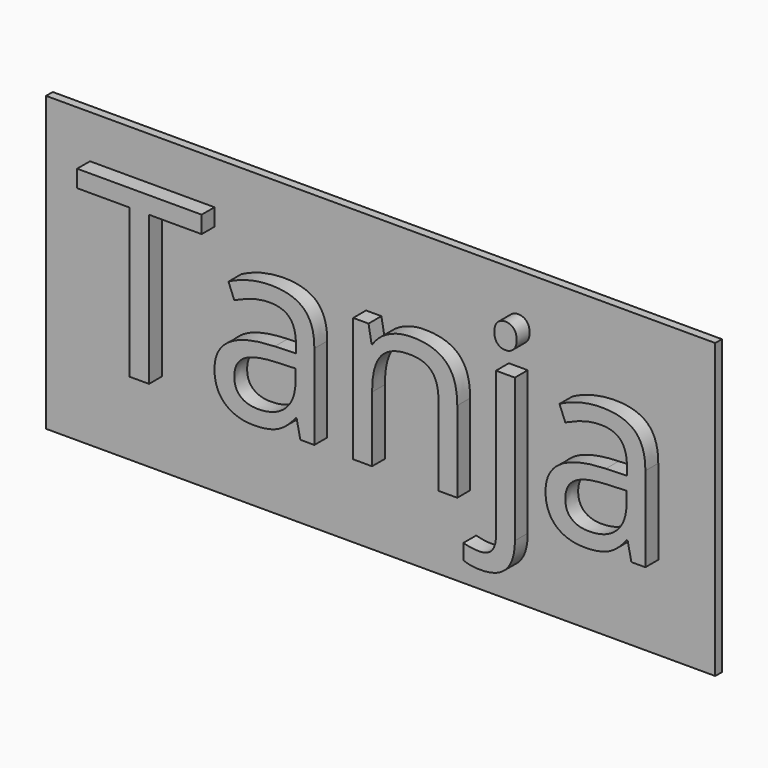
from build123d import *

# Parameters (mm, degrees)
F0_TEXT_SIZE = 27.7777777778
F1_DEPTH     = 2.920278348
F0_W         = 79.8914930556
F0_H         = 35
F2_DEPTH     = 1


# Not quite as in the source:
# - Text() gives the source's letters only with a copy of the font that has no kerning and outlines rounded to 1/6400 em; it was checked with that copy


with BuildPart() as f1:
    # F0 (on Front) → F1 (new body)
    with BuildSketch(Plane.XZ):
        with Locations((0, 0)):
            Text('Tanja', F0_TEXT_SIZE, font='Open Sans', text_align=(TextAlign.LEFT, TextAlign.BOTTOM))
    extrude(amount=F1_DEPTH)

    # F0 (on Front) → F2 (join)
    with BuildSketch(Plane.XZ):
        with Locations((34.9457465278, 7.5)):
            Rectangle(F0_W, F0_H)
        with BuildLine():
            Line((28.5677083333, 0), (26.8967013889, 0))
            Line((26.8967013889, 0), (26.4496527778, 2.1180555556))
            Line((26.4496527778, 2.1180555556), (26.3411458333, 2.1180555556))
            add(Edge.make_bspline(
                [(26.3411458333, 2.1180555556), (25.2300347222, 0.7204861111), (24.1254340278, 0.2235243056)],
                knots=[0, 0, 0, 1, 1, 1], degree=2))
            add(Edge.make_bspline(
                [(24.1254340278, 0.2235243056), (23.0208333333, -0.2734375), (21.3628472222, -0.2734375)],
                knots=[0, 0, 0, 1, 1, 1], degree=2))
            add(Edge.make_bspline(
                [(21.3628472222, -0.2734375), (19.1536458333, -0.2734375), (17.8993055556, 0.8680555556)],
                knots=[0, 0, 0, 1, 1, 1], degree=2))
            add(Edge.make_bspline(
                [(17.8993055556, 0.8680555556), (16.6449652778, 2.0095486111), (16.6449652778, 4.1102430556)],
                knots=[0, 0, 0, 1, 1, 1], degree=2))
            add(Edge.make_bspline(
                [(16.6449652778, 4.1102430556), (16.6449652778, 8.6111111111), (23.8454861111, 8.828125)],
                knots=[0, 0, 0, 1, 1, 1], degree=2))
            Line((23.8454861111, 8.828125), (26.3671875, 8.9105902778))
            Line((26.3671875, 8.9105902778), (26.3671875, 9.8350694444))
            add(Edge.make_bspline(
                [(26.3671875, 9.8350694444), (26.3671875, 11.5842013889), (25.6163194444, 12.4175347222)],
                knots=[0, 0, 0, 1, 1, 1], degree=2))
            add(Edge.make_bspline(
                [(25.6163194444, 12.4175347222), (24.8654513889, 13.2508680556), (23.2074652778, 13.2508680556)],
                knots=[0, 0, 0, 1, 1, 1], degree=2))
            add(Edge.make_bspline(
                [(23.2074652778, 13.2508680556), (21.3498263889, 13.2508680556), (19.0060763889, 12.1137152778)],
                knots=[0, 0, 0, 1, 1, 1], degree=2))
            Line((19.0060763889, 12.1137152778), (18.3116319444, 13.8368055556))
            add(Edge.make_bspline(
                [(18.3116319444, 13.8368055556), (19.4097222222, 14.4314236111), (20.7183159722, 14.7699652778)],
                knots=[0, 0, 0, 1, 1, 1], degree=2))
            add(Edge.make_bspline(
                [(20.7183159722, 14.7699652778), (22.0269097222, 15.1085069444), (23.3463541667, 15.1085069444)],
                knots=[0, 0, 0, 1, 1, 1], degree=2))
            add(Edge.make_bspline(
                [(23.3463541667, 15.1085069444), (26.0026041667, 15.1085069444), (27.28515625, 13.9301215278)],
                knots=[0, 0, 0, 1, 1, 1], degree=2))
            add(Edge.make_bspline(
                [(27.28515625, 13.9301215278), (28.5677083333, 12.7517361111), (28.5677083333, 10.1475694444)],
                knots=[0, 0, 0, 1, 1, 1], degree=2))
            Line((28.5677083333, 10.1475694444), (28.5677083333, 0))
        make_face(mode=Mode.SUBTRACT)
        with BuildLine():
            add(Edge.make_bspline(
                [(52.5043402778, -2.2786458333), (52.5043402778, -6.6753472222), (48.4461805556, -6.6753472222)],
                knots=[0, 0, 0, 1, 1, 1], degree=2))
            add(Edge.make_bspline(
                [(48.4461805556, -6.6753472222), (47.1571180556, -6.6753472222), (46.3585069444, -6.3324652778)],
                knots=[0, 0, 0, 1, 1, 1], degree=2))
            Line((46.3585069444, -6.3324652778), (46.3585069444, -4.5052083333))
            add(Edge.make_bspline(
                [(46.3585069444, -4.5052083333), (47.2960069444, -4.7743055556), (48.203125, -4.7743055556)],
                knots=[0, 0, 0, 1, 1, 1], degree=2))
            add(Edge.make_bspline(
                [(48.203125, -4.7743055556), (49.2621527778, -4.7743055556), (49.7569444444, -4.1970486111)],
                knots=[0, 0, 0, 1, 1, 1], degree=2))
            add(Edge.make_bspline(
                [(49.7569444444, -4.1970486111), (50.2517361111, -3.6197916667), (50.2517361111, -2.4435763889)],
                knots=[0, 0, 0, 1, 1, 1], degree=2))
            Line((50.2517361111, -2.4435763889), (50.2517361111, 14.8654513889))
            Line((50.2517361111, 14.8654513889), (52.5043402778, 14.8654513889))
            Line((52.5043402778, 14.8654513889), (52.5043402778, -2.2786458333))
        make_face(mode=Mode.SUBTRACT)
        with BuildLine():
            Line((68.0902777778, 0), (66.4192708333, 0))
            Line((66.4192708333, 0), (65.9722222222, 2.1180555556))
            Line((65.9722222222, 2.1180555556), (65.8637152778, 2.1180555556))
            add(Edge.make_bspline(
                [(65.8637152778, 2.1180555556), (64.7526041667, 0.7204861111), (63.6480034722, 0.2235243056)],
                knots=[0, 0, 0, 1, 1, 1], degree=2))
            add(Edge.make_bspline(
                [(63.6480034722, 0.2235243056), (62.5434027778, -0.2734375), (60.8854166667, -0.2734375)],
                knots=[0, 0, 0, 1, 1, 1], degree=2))
            add(Edge.make_bspline(
                [(60.8854166667, -0.2734375), (58.6762152778, -0.2734375), (57.421875, 0.8680555556)],
                knots=[0, 0, 0, 1, 1, 1], degree=2))
            add(Edge.make_bspline(
                [(57.421875, 0.8680555556), (56.1675347222, 2.0095486111), (56.1675347222, 4.1102430556)],
                knots=[0, 0, 0, 1, 1, 1], degree=2))
            add(Edge.make_bspline(
                [(56.1675347222, 4.1102430556), (56.1675347222, 8.6111111111), (63.3680555556, 8.828125)],
                knots=[0, 0, 0, 1, 1, 1], degree=2))
            Line((63.3680555556, 8.828125), (65.8897569444, 8.9105902778))
            Line((65.8897569444, 8.9105902778), (65.8897569444, 9.8350694444))
            add(Edge.make_bspline(
                [(65.8897569444, 9.8350694444), (65.8897569444, 11.5842013889), (65.1388888889, 12.4175347222)],
                knots=[0, 0, 0, 1, 1, 1], degree=2))
            add(Edge.make_bspline(
                [(65.1388888889, 12.4175347222), (64.3880208333, 13.2508680556), (62.7300347222, 13.2508680556)],
                knots=[0, 0, 0, 1, 1, 1], degree=2))
            add(Edge.make_bspline(
                [(62.7300347222, 13.2508680556), (60.8723958333, 13.2508680556), (58.5286458333, 12.1137152778)],
                knots=[0, 0, 0, 1, 1, 1], degree=2))
            Line((58.5286458333, 12.1137152778), (57.8342013889, 13.8368055556))
            add(Edge.make_bspline(
                [(57.8342013889, 13.8368055556), (58.9322916667, 14.4314236111), (60.2408854167, 14.7699652778)],
                knots=[0, 0, 0, 1, 1, 1], degree=2))
            add(Edge.make_bspline(
                [(60.2408854167, 14.7699652778), (61.5494791667, 15.1085069444), (62.8689236111, 15.1085069444)],
                knots=[0, 0, 0, 1, 1, 1], degree=2))
            add(Edge.make_bspline(
                [(62.8689236111, 15.1085069444), (65.5251736111, 15.1085069444), (66.8077256944, 13.9301215278)],
                knots=[0, 0, 0, 1, 1, 1], degree=2))
            add(Edge.make_bspline(
                [(66.8077256944, 13.9301215278), (68.0902777778, 12.7517361111), (68.0902777778, 10.1475694444)],
                knots=[0, 0, 0, 1, 1, 1], degree=2))
            Line((68.0902777778, 10.1475694444), (68.0902777778, 0))
        make_face(mode=Mode.SUBTRACT)
        Polygon((8.828125, 17.7821180556), (8.828125, 0), (6.5234375, 0), (6.5234375, 17.7821180556), (0.2430555556, 17.7821180556), (0.2430555556, 19.8307291667), (15.1085069444, 19.8307291667), (15.1085069444, 17.7821180556), align=None, mode=Mode.SUBTRACT)
        with BuildLine():
            Line((45.6293402778, 0), (43.3767361111, 0))
            Line((43.3767361111, 0), (43.3767361111, 9.6180555556))
            add(Edge.make_bspline(
                [(43.3767361111, 9.6180555556), (43.3767361111, 11.4322916667), (42.5499131944, 12.3285590278)],
                knots=[0, 0, 0, 1, 1, 1], degree=2))
            add(Edge.make_bspline(
                [(42.5499131944, 12.3285590278), (41.7230902778, 13.2248263889), (39.9565972222, 13.2248263889)],
                knots=[0, 0, 0, 1, 1, 1], degree=2))
            add(Edge.make_bspline(
                [(39.9565972222, 13.2248263889), (37.6258680556, 13.2248263889), (36.5407986111, 11.9639756944)],
                knots=[0, 0, 0, 1, 1, 1], degree=2))
            add(Edge.make_bspline(
                [(36.5407986111, 11.9639756944), (35.4557291667, 10.703125), (35.4557291667, 7.7994791667)],
                knots=[0, 0, 0, 1, 1, 1], degree=2))
            Line((35.4557291667, 7.7994791667), (35.4557291667, 0))
            Line((35.4557291667, 0), (33.203125, 0))
            Line((33.203125, 0), (33.203125, 14.8654513889))
            Line((33.203125, 14.8654513889), (35.0347222222, 14.8654513889))
            Line((35.0347222222, 14.8654513889), (35.3993055556, 12.8298611111))
            Line((35.3993055556, 12.8298611111), (35.5078125, 12.8298611111))
            add(Edge.make_bspline(
                [(35.5078125, 12.8298611111), (36.2022569444, 13.9279513889), (37.4500868056, 14.5334201389)],
                knots=[0, 0, 0, 1, 1, 1], degree=2))
            add(Edge.make_bspline(
                [(37.4500868056, 14.5334201389), (38.6979166667, 15.1388888889), (40.2300347222, 15.1388888889)],
                knots=[0, 0, 0, 1, 1, 1], degree=2))
            add(Edge.make_bspline(
                [(40.2300347222, 15.1388888889), (42.9166666667, 15.1388888889), (44.2730034722, 13.8433159722)],
                knots=[0, 0, 0, 1, 1, 1], degree=2))
            add(Edge.make_bspline(
                [(44.2730034722, 13.8433159722), (45.6293402778, 12.5477430556), (45.6293402778, 9.6961805556)],
                knots=[0, 0, 0, 1, 1, 1], degree=2))
            Line((45.6293402778, 9.6961805556), (45.6293402778, 0))
        make_face(mode=Mode.SUBTRACT)
        with BuildLine():
            add(Edge.make_bspline(
                [(50.4405381944, 17.7604166667), (50.0607638889, 18.1336805556), (50.0607638889, 18.8932291667)],
                knots=[0, 0, 0, 1, 1, 1], degree=2))
            add(Edge.make_bspline(
                [(50.0607638889, 18.8932291667), (50.0607638889, 19.6657986111), (50.4405381944, 20.0260416667)],
                knots=[0, 0, 0, 1, 1, 1], degree=2))
            add(Edge.make_bspline(
                [(50.4405381944, 20.0260416667), (50.8203125, 20.3862847222), (51.3932291667, 20.3862847222)],
                knots=[0, 0, 0, 1, 1, 1], degree=2))
            add(Edge.make_bspline(
                [(51.3932291667, 20.3862847222), (51.9357638889, 20.3862847222), (52.3285590278, 20.01953125)],
                knots=[0, 0, 0, 1, 1, 1], degree=2))
            add(Edge.make_bspline(
                [(52.3285590278, 20.01953125), (52.7213541667, 19.6527777778), (52.7213541667, 18.8932291667)],
                knots=[0, 0, 0, 1, 1, 1], degree=2))
            add(Edge.make_bspline(
                [(52.7213541667, 18.8932291667), (52.7213541667, 18.1336805556), (52.3285590278, 17.7604166667)],
                knots=[0, 0, 0, 1, 1, 1], degree=2))
            add(Edge.make_bspline(
                [(52.3285590278, 17.7604166667), (51.9357638889, 17.3871527778), (51.3932291667, 17.3871527778)],
                knots=[0, 0, 0, 1, 1, 1], degree=2))
            add(Edge.make_bspline(
                [(51.3932291667, 17.3871527778), (50.8203125, 17.3871527778), (50.4405381944, 17.7604166667)],
                knots=[0, 0, 0, 1, 1, 1], degree=2))
        make_face(mode=Mode.SUBTRACT)
        with BuildLine():
            add(Edge.make_bspline(
                [(59.2664930556, 2.2243923611), (60.0043402778, 1.5885416667), (61.3324652778, 1.5885416667)],
                knots=[0, 0, 0, 1, 1, 1], degree=2))
            add(Edge.make_bspline(
                [(61.3324652778, 1.5885416667), (63.4375, 1.5885416667), (64.6375868056, 2.7408854167)],
                knots=[0, 0, 0, 1, 1, 1], degree=2))
            add(Edge.make_bspline(
                [(64.6375868056, 2.7408854167), (65.8376736111, 3.8932291667), (65.8376736111, 5.9678819444)],
                knots=[0, 0, 0, 1, 1, 1], degree=2))
            Line((65.8376736111, 5.9678819444), (65.8376736111, 7.3090277778))
            Line((65.8376736111, 7.3090277778), (63.5850694444, 7.2178819444))
            add(Edge.make_bspline(
                [(63.5850694444, 7.2178819444), (60.8984375, 7.1223958333), (59.7135416667, 6.3823784722)],
                knots=[0, 0, 0, 1, 1, 1], degree=2))
            add(Edge.make_bspline(
                [(59.7135416667, 6.3823784722), (58.5286458333, 5.6423611111), (58.5286458333, 4.0842013889)],
                knots=[0, 0, 0, 1, 1, 1], degree=2))
            add(Edge.make_bspline(
                [(58.5286458333, 4.0842013889), (58.5286458333, 2.8602430556), (59.2664930556, 2.2243923611)],
                knots=[0, 0, 0, 1, 1, 1], degree=2))
        make_face()
        with BuildLine():
            add(Edge.make_bspline(
                [(19.7439236111, 2.2243923611), (20.4817708333, 1.5885416667), (21.8098958333, 1.5885416667)],
                knots=[0, 0, 0, 1, 1, 1], degree=2))
            add(Edge.make_bspline(
                [(21.8098958333, 1.5885416667), (23.9149305556, 1.5885416667), (25.1150173611, 2.7408854167)],
                knots=[0, 0, 0, 1, 1, 1], degree=2))
            add(Edge.make_bspline(
                [(25.1150173611, 2.7408854167), (26.3151041667, 3.8932291667), (26.3151041667, 5.9678819444)],
                knots=[0, 0, 0, 1, 1, 1], degree=2))
            Line((26.3151041667, 5.9678819444), (26.3151041667, 7.3090277778))
            Line((26.3151041667, 7.3090277778), (24.0625, 7.2178819444))
            add(Edge.make_bspline(
                [(24.0625, 7.2178819444), (21.3758680556, 7.1223958333), (20.1909722222, 6.3823784722)],
                knots=[0, 0, 0, 1, 1, 1], degree=2))
            add(Edge.make_bspline(
                [(20.1909722222, 6.3823784722), (19.0060763889, 5.6423611111), (19.0060763889, 4.0842013889)],
                knots=[0, 0, 0, 1, 1, 1], degree=2))
            add(Edge.make_bspline(
                [(19.0060763889, 4.0842013889), (19.0060763889, 2.8602430556), (19.7439236111, 2.2243923611)],
                knots=[0, 0, 0, 1, 1, 1], degree=2))
        make_face()
    extrude(amount=F2_DEPTH)


solid = f1.part
